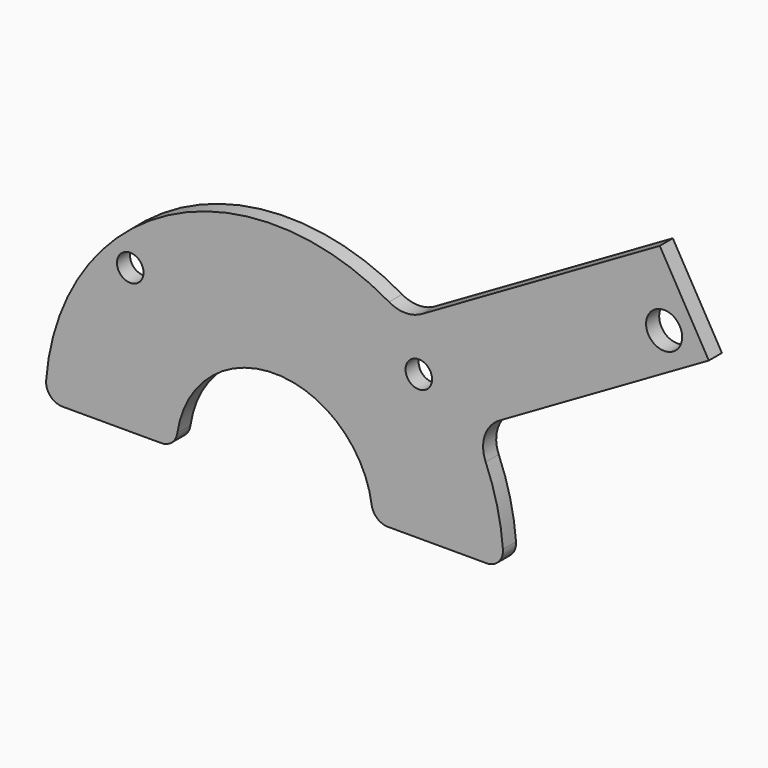
from build123d import *

# Parameters (mm, degrees)
F1_DEPTH = 6.35
F3_D     = 10.3124
F4_R     = 12.7
F5_R     = 6.35
F7_D     = 14


# Not quite as in the source:
# - a feature names something its author has since deleted; it is built from what else it names


with BuildPart() as f1:
    # F0 (on Front) → F1 (new body)
    with BuildSketch(Plane.XZ):
        with BuildLine():
            Line((38.1, 0), (88.9, 0))
            ThreePointArc((88.9, 0), (85.8708059571, 23.0090131096), (76.9896583964, 44.45))
            Line((76.9896583964, 44.45), (141.0511618856, 81.4359262841))
            Line((141.0511618856, 81.4359262841), (168.5474684557, 97.3109262841))
            Line((168.5474684557, 97.3109262841), (149.4974684557, 130.3064941683))
            Line((149.4974684557, 130.3064941683), (122.0011618856, 114.4314941683))
            Line((122.0011618856, 114.4314941683), (50.5107648032, 73.1564941683))
            ThreePointArc((50.5107648032, 73.1564941683), (-41.3086129578, 78.7198100576), (-88.9, 0))
            Line((-88.9, 0), (-38.1, 0))
            ThreePointArc((-38.1, 0), (0, 38.1), (38.1, 0))
        make_face()
    extrude(amount=F1_DEPTH)

    # F3 (through all)
    with Locations(Plane.XZ.offset(6.35)):
        with Locations((-55.9918969149, 55.9918969149), (55.9918969149, 55.9918969149)):
            Hole(F3_D / 2)

    # F4
    f4_edges = [f1.edges().sort_by_distance(p)[0] for p in [
        (50.510765, -3.175, 73.156494),
        (76.989658, -3.175, 44.45),
    ]]
    fillet(f4_edges, radius=F4_R)

    # F5
    f5_edges = [f1.edges().sort_by_distance(p)[0] for p in [
        (88.9, -3.175, 0),
        (38.1, -3.175, 0),
        (-38.1, -3.175, 0),
        (-88.9, -3.175, 0),
    ]]
    fillet(f5_edges, radius=F5_R)

    # F7 (through all)
    with Locations(Plane.XZ.offset(6.35)):
        with Locations((151.1989458277, 101.9594489122)):
            Hole(F7_D / 2)


solid = f1.part
